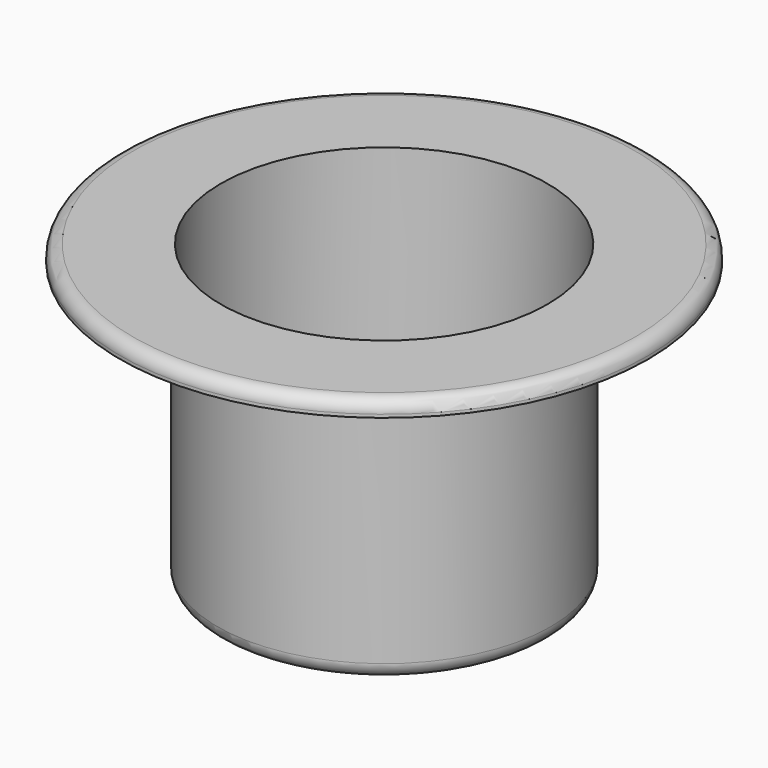
from build123d import *

# Parameters (mm, degrees)
F0_R     = 42
F0_R_2   = 26
F1_DEPTH = 2.5
F2_R     = 2
F3_R     = 26.5
F4_DEPTH = 45
F5_R     = 2.5
F6_T     = -0.5


# Not quite as in the source:
# - a shell that OpenCascade refuses in one call is made with other operations: the cavity is built on its own and cut out


with BuildPart() as f1:
    # F0 (on Top) → F1 (new body)
    with BuildSketch(Plane.XY):
        Circle(F0_R)
        Circle(F0_R_2, mode=Mode.SUBTRACT)
    extrude(amount=F1_DEPTH)

    # F2
    f2_edges = [f1.edges().sort_by_distance(p)[0] for p in [
        (-42, 0, 2.5),
    ]]
    fillet(f2_edges, radius=F2_R)

    # F3 (on face) → F4 (join)
    with BuildSketch(Plane(origin=(0, 0, 0), x_dir=(1, 0, 0), z_dir=(0, 0, -1))):
        Circle(F3_R)
    extrude(amount=F4_DEPTH)

    # F5
    f5_edges = [f1.edges().sort_by_distance(p)[0] for p in [
        (-26.5, 0, -45),
    ]]
    fillet(f5_edges, radius=F5_R)

    # F6: a shell. OpenCascade refuses it in one call, so the cavity is built on its own and cut out:
    # the body offset inwards by the wall thickness, plus a prism from it out through each open face.
    f6_core = offset(f1.part, amount=F6_T, kind=Kind.INTERSECTION, mode=Mode.PRIVATE)
    f6_exits = [f6_core.faces().sort_by_distance(p)[0] for p in [
        (0, 0, -0.5),
    ]]
    add(f6_core, mode=Mode.SUBTRACT)
    extrude(f6_exits, amount=-F6_T, mode=Mode.SUBTRACT)


solid = f1.part
